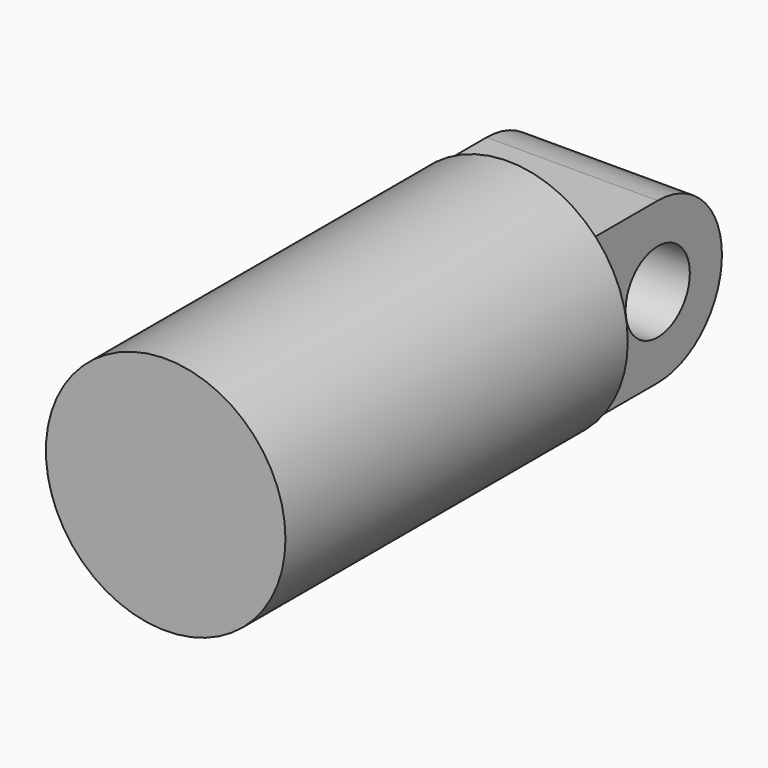
from build123d import *

# Parameters (mm, degrees)
F0_R     = 14.224
F1_DEPTH = 50.8
F2_W     = 19.05
F2_H     = 19.05
F3_DEPTH = 10.16
F4_R     = 4.7625
F5_DEPTH = 25.4
F6_R     = 9.52499


# Not quite as in the source:
# - a fillet or chamfer is up to 0.001 mm smaller than in the source, because OpenCascade refuses the exact size


with BuildPart() as f1:
    # F0 (on Front) → F1 (new body)
    with BuildSketch(Plane.XZ):
        Circle(F0_R)
    extrude(amount=F1_DEPTH)

    # F2 (on Right) → F3 (join, symmetric)
    with BuildSketch(Plane.YZ):
        with Locations((9.525, 0)):
            Rectangle(F2_W, F2_H)
    extrude(amount=F3_DEPTH, both=True)

    # F4 (on face) → F5 (cut)
    with BuildSketch(Plane.YZ.offset(10.16)):
        with Locations((9.525, 0)):
            Circle(F4_R)
    extrude(amount=-F5_DEPTH, mode=Mode.SUBTRACT)

    # F6 (radius 9.525 in the source; OpenCascade refuses exactly that, so slightly less here)
    f6_edges = [f1.edges().sort_by_distance(p)[0] for p in [
        (0, 19.05, 9.525),
        (0, 19.05, -9.525),
    ]]
    fillet(f6_edges, radius=F6_R)


solid = f1.part
